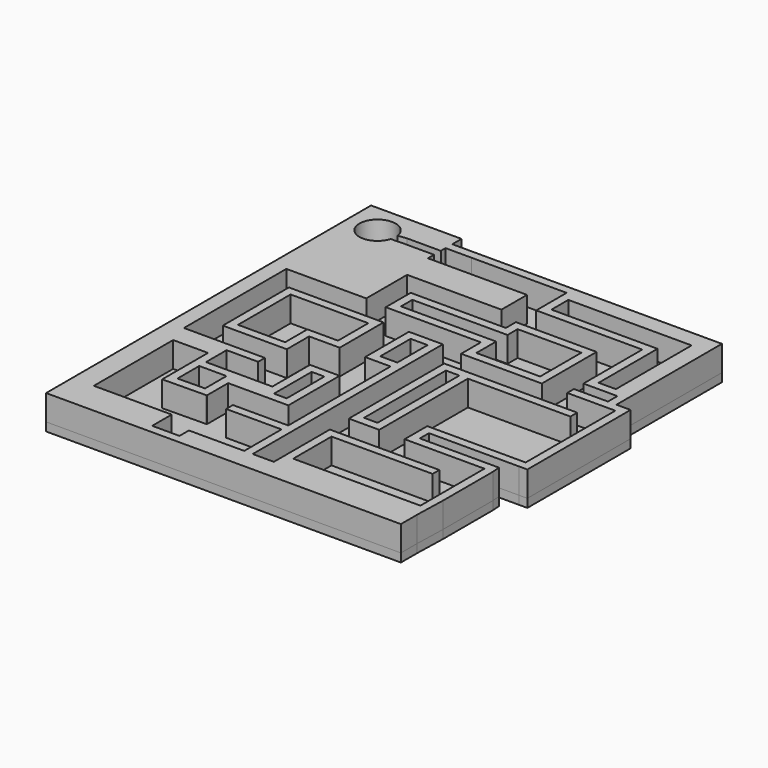
from build123d import *

# Parameters (mm, degrees)
F0_W     = 4.0089304447
F0_H     = 8.9445743561
F0_W_2   = 3.0044652224
F0_H_2   = 11.1408379897
F0_W_3   = 6.445730105
F0_H_3   = 1.9999999106
F1_DEPTH = 6
F0_W_4   = 3.187499553
F0_H_4   = 24.1854941323
F3_DEPTH = 2


# Not quite as in the source:
# - ends of sketch curves that miss each other by under 0.0002 mm in the source are joined
# - a feature names something its author has since deleted; it is built from what else it names


with BuildPart() as f1:
    # F0 (on Top) → F1 (new body)
    with BuildSketch(Plane.XY):
        Polygon((33.8502417803, -48), (35.8502417803, -48), (35.8502417803, -43.2157492936), (2, -43.2157492936), (-3, -43.2157492936), (-5, -43.2157492936), (-10.0380338952, -43.2157492936), (-18.0760677904, -43.2157492936), (-18.0760677904, -46.0000000894), (-18.0760677904, -48), (-16.0760677904, -48), (-16.0760677904, -45.2157492936), (2, -45.2157492936), (33.8502417803, -45.2157492936), align=None)
        with BuildLine():
            Line((2, -43.2157492936), (35.8502417803, -43.2157492936))
            Line((35.8502417803, -43.2157492936), (36.050270915, -35.7734388411))
            Line((36.050270915, -35.7734388411), (36.050270915, -26.6810520291))
            Line((36.050270915, -26.6810520291), (36.050270915, -21.0760677904))
            Line((36.050270915, -21.0760677904), (35.9028056264, -19.0760677904))
            Line((35.9028056264, -19.0760677904), (34.050270915, -19.0760677904))
            Line((34.050270915, -19.0760677904), (17.187499553, -19.0760677904))
            Line((17.187499553, -19.0760677904), (17.187499553, -16.3839283586))
            Line((17.187499553, -16.3839283586), (38.4385609329, -16.3839283586))
            Line((38.4385609329, -16.3839283586), (40.4385609329, -16.3751612157))
            Line((40.4385609329, -16.3751612157), (40.4385609329, -14.3839283586))
            Line((40.4385609329, -14.3839283586), (40.4385609329, 3.685426342))
            Line((40.4385609329, 3.685426342), (40.4385609329, 12.109426342))
            Line((40.4385609329, 12.109426342), (40.4385609329, 14.109426342))
            Line((40.4385609329, 14.109426342), (37.0984218628, 14.109426342))
            Line((37.0984218628, 14.109426342), (37.0984218628, 16.9020142178))
            Line((37.0984218628, 16.9020142178), (37.0984218628, 45.2713289261))
            Line((37.0984218628, 45.2713289261), (34.151788801, 45.2713289261))
            Line((34.151788801, 45.2713289261), (15.1339303702, 45.2713289261))
            Line((15.1339303702, 45.2713289261), (12.723213993, 45.2713289261))
            Line((12.723213993, 45.2713289261), (2, 45.2713289261))
            Line((2, 45.2713289261), (-20.491072908, 45.2713289261))
            Line((-20.491072908, 45.2713289261), (-26.6181714833, 45.2713289261))
            Line((-26.6181714833, 45.2713289261), (-26.6181714833, 48))
            Line((-26.6181714833, 48), (-28.6181714833, 48))
            Line((-28.6181714833, 48), (-28.6181714833, 43.2713292539))
            Line((-28.6181714833, 43.2713292539), (-35.0209371383, 43.2713292539))
            ThreePointArc((-35.0209371383, 43.2713292539), (-47.1567057037, 41.4034289905), (-35.3387935174, 38.0713303089))
            Line((-35.3387935174, 38.0713303089), (-28.6181714833, 38.0713303089))
            Line((-28.6181714833, 38.0713303089), (-28.6181714833, 36.0713303089))
            Line((-28.6181714833, 36.0713303089), (-5.1999986172, 36.0713303089))
            Line((-5.1999986172, 36.0713303089), (-5.1999986172, 32.5106177479))
            Line((-5.1999986172, 32.5106177479), (-27.4899210781, 32.5106177479))
            Line((-27.4899210781, 32.5106177479), (-27.4899210781, 25.3106191307))
            Line((-27.4899210781, 25.3106191307), (-27.4899210781, 20.4432241027))
            Line((-27.4899210781, 20.4432241027), (-44.3228720746, 20.4432241027))
            Line((-44.3228720746, 20.4432241027), (-46.375002712, 20.4654708505))
            Line((-46.375002712, 20.4654708505), (-46.375002712, 18.4439036259))
            Line((-46.375002712, 18.4439036259), (-46.375002712, -13.5858533904))
            Line((-46.375002712, -13.5858533904), (-46.375002712, -44.2410755157))
            Line((-46.375002712, -44.2410755157), (-26.5217978954, -44.2410755157))
            Line((-26.5217978954, -44.2410755157), (-24.5217978954, -44.2410755157))
            Line((-24.5217978954, -44.2410755157), (-24.5217978954, -43.2354741863))
            Line((-24.5217978954, -43.2354741863), (-24.5217978954, -42.2410755157))
            Line((-24.5217978954, -42.2410755157), (-44.919644922, -42.2410755157))
            Line((-44.919644922, -42.2410755157), (-44.919644922, -35.2232158184))
            Line((-44.919644922, -35.2232158184), (-44.919644922, -14.8125016391))
            Line((-44.919644922, -14.8125016391), (-44.919644922, -13.8125016391))
            Line((-44.919644922, -13.8125016391), (-34.687500447, -13.8125016391))
            Line((-34.687500447, -13.8125016391), (-32.687500447, -13.8125016391))
            Line((-32.687500447, -13.8125016391), (-25.2415498942, -13.8125016391))
            Line((-25.2415498942, -13.8125016391), (-25.2415498942, -11.812501587))
            Line((-25.2415498942, -11.812501587), (-44.3750029793, -11.812501587))
            Line((-44.3750029793, -11.812501587), (-44.3750029793, -11.5858536577))
            Line((-44.3750029793, -11.5858536577), (-44.3750029793, 18.4439036259))
            Line((-44.3750029793, 18.4439036259), (-25.4899210781, 18.4439036259))
            Line((-25.4899210781, 18.4439036259), (-25.4899210781, 25.3106191307))
            Line((-25.4899210781, 25.3106191307), (-25.4899210781, 30.5106177479))
            Line((-25.4899210781, 30.5106177479), (-3.1999986172, 30.5106177479))
            Line((-3.1999986172, 30.5106177479), (-3.1999986172, 38.0713303089))
            Line((-3.1999986172, 38.0713303089), (-26.6181714833, 38.0713303089))
            Line((-26.6181714833, 38.0713303089), (-26.6181714833, 39.1947031021))
            Line((-26.6181714833, 39.1947031021), (-26.6181714833, 39.8743376136))
            Line((-26.6181714833, 39.8743376136), (-28.6181714833, 39.8743376136))
            Line((-28.6181714833, 39.8743376136), (-34.662083278, 39.8743376136))
            Line((-34.662083278, 39.8743376136), (-36.7890999075, 39.7738576335))
            ThreePointArc((-36.7890999075, 39.7738576335), (-45.1548993555, 41.3600169533), (-36.6435097314, 41.6023977682))
            Line((-36.6435097314, 41.6023977682), (-34.662083278, 41.8743377626))
            Line((-34.662083278, 41.8743377626), (-28.6181714833, 41.8743377626))
            Line((-28.6181714833, 41.8743377626), (-26.6175400466, 41.8743377626))
            Line((-26.6175400466, 41.8743377626), (-26.6181714833, 41.9328399003))
            Line((-26.6181714833, 41.9328399003), (-26.6181714833, 43.2713292539))
            Line((-26.6181714833, 43.2713292539), (-20.491072908, 43.2713292539))
            Line((-20.491072908, 43.2713292539), (2, 43.2713289261))
            Line((2, 43.2713289261), (2, 34.2909740284))
            Line((2, 34.2909740284), (27.0624984726, 34.2909740284))
            Line((27.0624984726, 34.2909740284), (27.0624984726, 16.9017884657))
            Line((27.0624984726, 16.9017884657), (35.0984223187, 16.9017884657))
            Line((35.0984223187, 16.9017884657), (35.0984223187, 14.109426342))
            Line((35.0984223187, 14.109426342), (27.0624984726, 14.109426342))
            Line((27.0624984726, 14.109426342), (27.0624984726, 12.109426342))
            Line((27.0624984726, 12.109426342), (35.1339298114, 12.109426342))
            Line((35.1339298114, 12.109426342), (37.0984218628, 12.109426342))
            Line((37.0984218628, 12.109426342), (38.4385609329, 12.109426342))
            Line((38.4385609329, 12.109426342), (38.4385609329, 3.685426342))
            Line((38.4385609329, 3.685426342), (38.4385609329, -14.3839283586))
            Line((38.4385609329, -14.3839283586), (15.187499553, -14.3839283586))
            Line((15.187499553, -14.3839283586), (15.187499553, -21.0760677904))
            Line((15.187499553, -21.0760677904), (34.050270915, -21.0760677904))
            Line((34.050270915, -21.0760677904), (34.050270915, -26.6810520291))
            Line((34.050270915, -26.6810520291), (34.050270915, -35.7734388411))
            Line((34.050270915, -35.7734388411), (34.050270915, -39.9928833097))
            Line((34.050270915, -39.9928833097), (4.00000019, -39.9928833097))
            Line((4.00000019, -39.9928833097), (4.00000019, -28.6810520291))
            Line((4.00000019, -28.6810520291), (27.8847850859, -28.6810520291))
            Line((27.8847850859, -28.6810520291), (27.8847850859, -26.6810520291))
            Line((27.8847850859, -26.6810520291), (2, -26.6810520291))
            Line((2, -26.6810520291), (2, -43.2157492936))
        make_face()
        Polygon((29.0624984726, 36.2909740284), (7, 36.2909740284), (4, 36.2909740284), (4, 41.2713289261), (12.723213993, 41.2713289261), (15.1339303702, 41.2713289261), (33.1339298114, 41.2713289261), (33.1339298114, 18.9017884657), (29.0624984726, 18.9017884657), align=None, mode=Mode.SUBTRACT)
        Polygon((-5, 0), (-3, 0), (-3, 12.9445743561), (-5, 12.9445743561), (-11.0089304447, 12.9445743561), (-11.0089304447, 0), align=None)
        with Locations((-7.0044652224, 6.472287178)):
            Rectangle(F0_W, F0_H, mode=Mode.SUBTRACT)
        Polygon((-5, -30.2095213234), (-3, -30.2095213234), (-3, -2.745107308), (-3, 0), (-5, 0), (-5, -2.745107308), align=None)
        Polygon((-32.687500447, -19.9017883539), (-34.687500447, -19.9017883539), (-34.687500447, -30.3482176065), (-24.5217978954, -30.2095213234), (-24.2415498942, -30.1899854094), (-24.2415498942, -24.0735206753), (-24.2415498942, -23.9196424633), (-10.0044652224, -23.9196424633), (-10.0044652224, -8.7788044736), (-17.0089304447, -8.7788044736), (-17.0089304447, -14.8125016391), (-17.0089304447, -19.9017883539), align=None)
        Polygon((-26.4358265479, -28.2354493335), (-32.687500447, -28.3207443663), (-32.687500447, -21.9017883539), (-26.2415498942, -21.9017883539), (-26.2605734169, -23.9196424633), (-26.2415498942, -24.0735206753), (-26.2415498942, -28.2354493335), align=None, mode=Mode.SUBTRACT)
        with Locations((-13.5066978335, -16.3492234685)):
            Rectangle(F0_W_2, F0_H_2, mode=Mode.SUBTRACT)
        Polygon((-44.919644922, -42.2410755157), (-24.5217978954, -42.2410755157), (-24.5217978954, -40.2410755157), (-42.919644922, -40.2410755157), (-42.919644922, -35.2232158184), (-42.919644922, -16.8125016391), (-34.687500447, -16.8125016391), (-34.687500447, -14.8125016391), (-34.687500447, -13.8125016391), (-44.919644922, -13.8125016391), (-44.919644922, -14.8125016391), (-44.919644922, -35.2232158184), align=None)
        Polygon((-32.687500447, -13.8125016391), (-34.687500447, -13.8125016391), (-34.687500447, -14.8125016391), (-34.687500447, -16.8125016391), (-34.687500447, -19.9017883539), (-32.687500447, -19.9017883539), (-32.687500447, -14.8125016391), align=None)
        Polygon((-5, -43.2157492936), (-3, -43.2157492936), (-3, -30.2095213234), (-5, -30.2095213234), (-8.0380338952, -30.2095213234), (-18.0803574622, -30.2095213234), (-18.0803574622, -32.2095213234), (-10.0380338952, -32.2095213234), (-8.0380338952, -32.2095213234), (-5, -32.2095213234), align=None)
        Polygon((-16.0760677904, -48), (33.8502417803, -48), (33.8502417803, -45.2157492936), (2, -45.2157492936), (-16.0760677904, -45.2157492936), align=None)
        with BuildLine():
            Line((-28.6181714833, 43.2713292539), (-28.6181714833, 48))
            Line((-28.6181714833, 48), (-48, 48))
            Line((-48, 48), (-48, -48))
            Line((-48, -48), (-26.5217982233, -48))
            Line((-26.5217982233, -48), (-26.5217982233, -44.2410755157))
            Line((-26.5217982233, -44.2410755157), (-46.375002712, -44.2410755157))
            Line((-46.375002712, -44.2410755157), (-46.375002712, -13.5858533904))
            Line((-46.375002712, -13.5858533904), (-46.375002712, 18.4439036259))
            Line((-46.375002712, 18.4439036259), (-46.375002712, 20.4654708505))
            Line((-46.375002712, 20.4654708505), (-44.3228720746, 20.4432241027))
            Line((-44.3228720746, 20.4432241027), (-27.4899210781, 20.4432241027))
            Line((-27.4899210781, 20.4432241027), (-27.4899210781, 25.3106191307))
            Line((-27.4899210781, 25.3106191307), (-27.4899210781, 32.5106177479))
            Line((-27.4899210781, 32.5106177479), (-5.1999986172, 32.5106177479))
            Line((-5.1999986172, 32.5106177479), (-5.1999986172, 36.0713303089))
            Line((-5.1999986172, 36.0713303089), (-28.6181714833, 36.0713303089))
            Line((-28.6181714833, 36.0713303089), (-28.6181714833, 38.0713303089))
            Line((-28.6181714833, 38.0713303089), (-35.3387935174, 38.0713303089))
            ThreePointArc((-35.3387935174, 38.0713303089), (-47.1567057037, 41.4034289905), (-35.0209371383, 43.2713292539))
            Line((-35.0209371383, 43.2713292539), (-28.6181714833, 43.2713292539))
        make_face()
        with Locations((-21.2989328429, -47.0000000447)):
            Rectangle(F0_W_3, F0_H_3)
        Polygon((-26.5217982233, -48), (-24.5217978954, -48), (-24.5217978954, -46.0000000894), (-24.5217978954, -44.2410755157), (-26.5217978954, -44.2410755157), align=None)
    extrude(amount=F1_DEPTH)


with BuildPart() as f1b:
    # F0 (on Top) → F1, piece 2 (new body)
    with BuildSketch(Plane.XY):
        Polygon((-17.0089304447, 12.9445743561), (-25.2899224609, 12.9445743561), (-25.3159923449, 12.9445744678), (-37.3750032112, 12.9445744678), (-39.3750034273, 12.9445744678), (-39.3750034273, -6.5858541057), (-28.7255346775, -6.5858541057), (-24.2415498942, -6.5858541057), (-24.2415498942, -2.745107308), (-24.2415498942, 0), (-17.0089304447, 0), align=None)
        Polygon((-28.7255346775, -4.5858538896), (-37.3750032112, -4.5858538896), (-37.3750032112, 10.94457414), (-25.3159923449, 10.94457414), (-19.0089306608, 10.94457414), (-19.0089306608, 2.0000002161), (-26.2415501103, 2.0000002161), (-26.2415501103, -2.745107308), (-26.2415501103, -4.5858538896), align=None, mode=Mode.SUBTRACT)
    extrude(amount=F1_DEPTH)


with BuildPart() as f1c:
    # F0 (on Top) → F1, piece 3 (new body)
    with BuildSketch(Plane.XY):
        Polygon((2, 28.2909740284), (2, 25.3106191307), (-20.4899210781, 25.3106191307), (-20.4899210781, 17.9445743561), (-18.4899210781, 17.9445743561), (-2.5132134371, 17.9445743561), (2, 17.9445743561), (2, 12.109426342), (21.0624984726, 12.109426342), (21.0624984726, 28.2909740284), align=None)
        Polygon((-2.5132134371, 19.9445743561), (-18.4899210781, 19.9445743561), (-18.4899210781, 23.3106191307), (4, 23.3106191307), (4, 26.2909740284), (19.0624984726, 26.2909740284), (19.0624984726, 22.2909741402), (19.0624984726, 14.109426342), (4, 14.109426342), (4, 19.9445743561), align=None, mode=Mode.SUBTRACT)
    extrude(amount=F1_DEPTH)


with BuildPart() as f1d:
    # F0 (on Top) → F1, piece 4 (new body)
    with BuildSketch(Plane.XY):
        Polygon((4, 7.1094264276), (2, 7.109426342), (2, -21.0760677904), (9.187499553, -21.0760677904), (9.187499553, 5.109426342), (15.187499553, 5.109426342), (17.187499553, 5.109426342), (28.4385609925, 5.109426342), (30.4385609925, 5.109426342), (33.4385609925, 5.109426342), (33.4385609925, 7.1094264276), (30.4385609925, 7.1094264276), (9.187499553, 7.1094264276), (7.187499553, 7.1094264276), align=None)
        with Locations((5.5937497765, -6.9833207242)):
            Rectangle(F0_W_4, F0_H_4, mode=Mode.SUBTRACT)
    extrude(amount=F1_DEPTH)


with BuildPart() as f3:
    # F2 (on face) → F3 (new body)
    with BuildSketch(Plane(origin=(0, 0, 0), x_dir=(1, 0, 0), z_dir=(0, 0, -1))):
        Polygon((35.8502417803, 48), (-48, 48), (-48, -48), (-26.6181714833, -48), (-26.6181714833, -45.2713289261), (37.0984218628, -45.2713289261), (37.0984218628, -14.109426342), (40.4385609329, -14.109426342), (40.4385609329, 16.3751612157), (38.4385609329, 16.3839283586), (17.187499553, 16.3839283586), (17.187499553, 19.0760677904), (35.9028056264, 19.0760677904), (36.050270915, 21.0760677904), (36.050270915, 35.7734388411), (35.8502417803, 43.2157492936), align=None)
    extrude(amount=F3_DEPTH)


solid = Compound([f1.part, f1b.part, f1c.part, f1d.part, f3.part])
